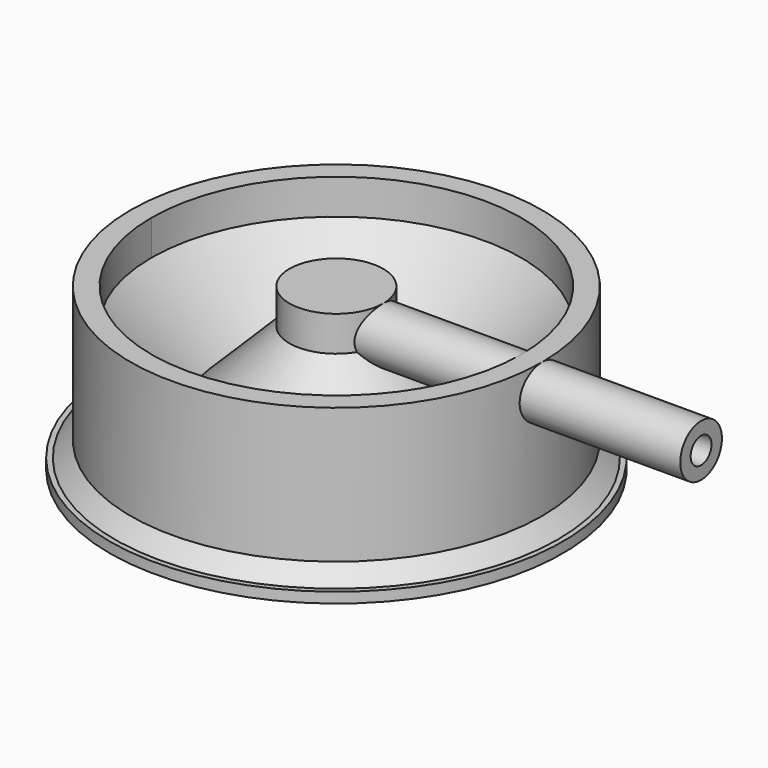
from build123d import *

# Parameters (mm, degrees)
F2_SIZE2      = 1.5
F2_SIZE       = 1.5
F7_END_RADIUS = 4.5
F6_R          = 2.5
F6_R_2        = 1.25
F7_REACH      = 53.8220678119
F8_DEPTH      = 27.5
F9_DEPTH      = 10


with BuildPart() as f1:
    # F0 (on Front) → F1 (revolve)
    with BuildSketch(Plane.XZ):
        Polygon((-21.75, 1), (-21.75, 0), (-19.75, -0.7279404685), (-2.5, 2.3136999487), (-2.5, 3.5), (-19.75, 3.5), (-19.75, 1), align=None)
    revolve(axis=Axis((0, 0, 1.1568499743), (0, 0, -1)))

    # F2
    f2_edges = [f1.edges().sort_by_distance(p)[0] for p in [
        (19.75, 0, 1),
    ]]
    chamfer(f2_edges, length=F2_SIZE, length2=F2_SIZE2)

    # F3 (on Front) → F4 (revolve)
    with BuildSketch(Plane.XZ):
        Polygon((-19.75, 15.5), (-19.75, 3.5), (-2.5, 3.5), (-2.5, 13.5), (0, 13.5), (0, 15.5), (-4.5, 15.5), (-4.5, 12.125), (-11.125, 5.5), (-17.75, 12.125), (-17.75, 15.5), align=None)
    revolve(axis=Axis((0, 0, 14.5), (0, 0, -1)))

    f7_end = (Plane(origin=(0, 0, 13.8125), x_dir=(-1, 0, 0), z_dir=(0, 0, -1)) * Cylinder(F7_END_RADIUS, 234.8895057061, mode=Mode.PRIVATE)).faces().sort_by_distance((4.5, 0, 13.8125))[0]
    # F6 (on offset) → F7 (join, up to the whole of a round face its end follows)
    with BuildSketch(Plane.YZ.offset(25)):
        with Locations((0, 13)):
            Circle(F6_R)
        with Locations((0, 13)):
            Circle(F6_R_2, mode=Mode.SUBTRACT)
        with Locations((0, 13)):
            Circle(F6_R_2)
    f7_long = extrude(amount=-F7_REACH, mode=Mode.PRIVATE)
    add(split(f7_long, bisect_by=f7_end, keep=Keep.ALL, mode=Mode.PRIVATE).solids().sort_by_distance((25, 0, 13))[0])

    # F6 (on offset) → F8 (cut)
    with BuildSketch(Plane.YZ.offset(25)):
        with Locations((0, 13)):
            Circle(F6_R_2)
    extrude(amount=-F8_DEPTH, mode=Mode.SUBTRACT)

    # F6 (on offset) → F9 (join)
    with BuildSketch(Plane.YZ.offset(25)):
        with Locations((0, 13)):
            Circle(F6_R)
        with Locations((0, 13)):
            Circle(F6_R_2, mode=Mode.SUBTRACT)
    extrude(amount=F9_DEPTH)


solid = f1.part
